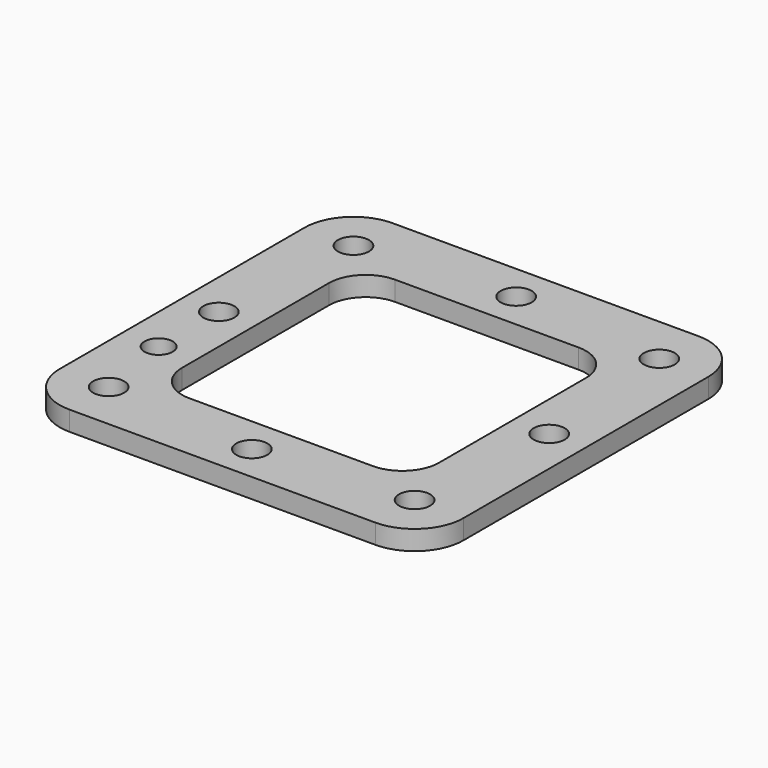
from build123d import *

# Parameters (mm, degrees)
F1_DEPTH = 8
F2_R     = 6.35
F3_DEPTH = 8.001
F4_D     = 11.50874


with BuildPart() as f1:
    # F0 (on Top) → F1 (new body)
    with BuildSketch(Plane.XY):
        with BuildLine():
            Line((31.3706356287, 124.5844857395), (-93.6293643713, 124.5844857395))
            ThreePointArc((-93.6293643713, 124.5844857395), (-107.771499995, 118.7266213632), (-113.6293643713, 104.5844857395))
            Line((-113.6293643713, 104.5844857395), (-113.6293643713, -20.4155142605))
            ThreePointArc((-113.6293643713, -20.4155142605), (-107.771499995, -34.5576498843), (-93.6293643713, -40.4155142605))
            Line((-93.6293643713, -40.4155142605), (31.3706356287, -40.4155142605))
            ThreePointArc((31.3706356287, -40.4155142605), (45.5127712524, -34.5576498843), (51.3706356287, -20.4155142605))
            Line((51.3706356287, -20.4155142605), (51.3706356287, 104.5844857395))
            ThreePointArc((51.3706356287, 104.5844857395), (45.5127712524, 118.7266213632), (31.3706356287, 124.5844857395))
        make_face()
        with BuildLine():
            ThreePointArc((-83.6293643713, 79.5844857395), (-79.2359660891, 90.1910874573), (-68.6293643713, 94.5844857395))
            Line((-68.6293643713, 94.5844857395), (6.3706356287, 94.5844857395))
            ThreePointArc((6.3706356287, 94.5844857395), (16.9772373465, 90.1910874573), (21.3706356287, 79.5844857395))
            Line((21.3706356287, 79.5844857395), (21.3706356287, 4.5844857395))
            ThreePointArc((21.3706356287, 4.5844857395), (16.9772373465, -6.0221159783), (6.3706356287, -10.4155142605))
            Line((6.3706356287, -10.4155142605), (-68.6293643713, -10.4155142605))
            ThreePointArc((-68.6293643713, -10.4155142605), (-79.2359660891, -6.0221159783), (-83.6293643713, 4.5844857395))
            Line((-83.6293643713, 4.5844857395), (-83.6293643713, 79.5844857395))
        make_face(mode=Mode.SUBTRACT)
    extrude(amount=F1_DEPTH)

    # F2 (on face) → F3 (cut, through all)
    with BuildSketch(Plane.XY.offset(8)):
        with Locations((-93.6293643713, 104.5844857395)):
            Circle(F2_R)
        with Locations((-31.1293643713, 109.5844857395)):
            Circle(F2_R)
        with Locations((31.3706356287, 104.5844857395)):
            Circle(F2_R)
        with Locations((36.3706356287, 42.0844857395)):
            Circle(F2_R)
        with Locations((31.3706356287, -20.4155142605)):
            Circle(F2_R)
        with Locations((-31.1293643713, -25.4155142605)):
            Circle(F2_R)
        with Locations((-93.6293643713, -20.4155142605)):
            Circle(F2_R)
        with Locations((-98.6293643713, 42.0844857395)):
            Circle(F2_R)
    extrude(amount=-F3_DEPTH, mode=Mode.SUBTRACT)

    # F4 (through all)
    with Locations(Plane.XY.offset(8)):
        with Locations((-98.6293643713, 11.3532003015)):
            Hole(F4_D / 2)


solid = f1.part
